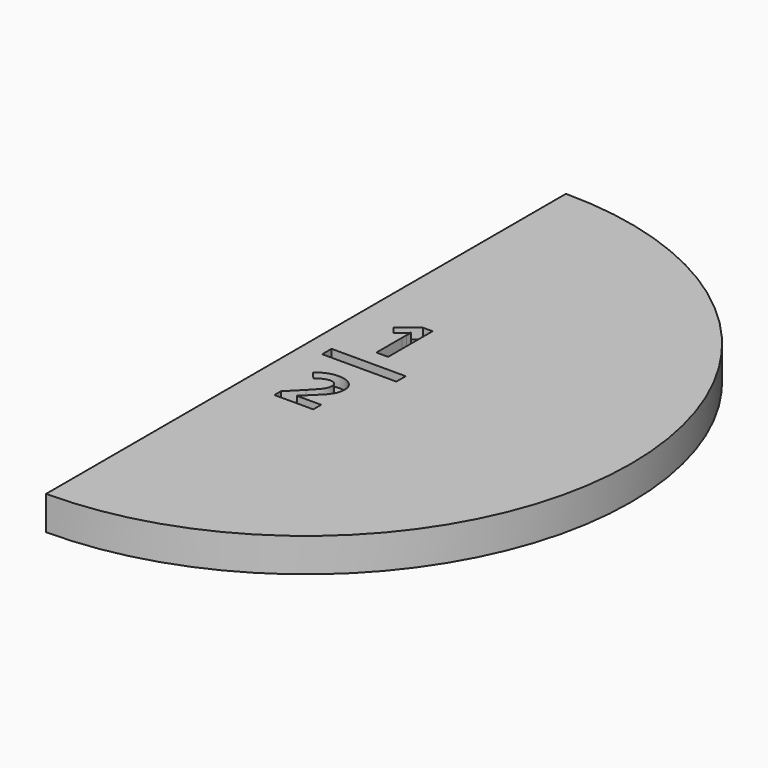
from build123d import *

# Parameters (mm, degrees)
F1_DEPTH      = 6.5
F2_R          = 12.5
F6_DEPTH      = 5
F3_R          = 12.5
F7_DEPTH      = 5
F4_R          = 12.5
F8_DEPTH      = 5
F5_R          = 12.5
F9_DEPTH      = 5
F10_W         = 14.2726595514
F10_H         = 2.253577346
F11_DEPTH     = 2
F15_TEXT_SIZE = 14.9677896982
F16_DEPTH     = 2


# Not quite as in the source:
# - Text() gives the source's letters only with a copy of the font that has no kerning and outlines rounded to 1/6400 em; it was checked with that copy


with BuildPart() as f1:
    # F0 (on Top) → F1 (new body)
    with BuildSketch(Plane.XY):
        with BuildLine():
            Line((0, 62.5), (0, -62.5))
            ThreePointArc((0, -62.5), (62.5, 0), (0, 62.5))
        make_face()
    extrude(amount=F1_DEPTH)

    # F2 (on face) → F6 (cut)
    with BuildSketch(Plane.XY.offset(6.5)):
        with Locations((17.2774232924, 41.4407812059)):
            Circle(F2_R)
    extrude(amount=-F6_DEPTH, mode=Mode.SUBTRACT)

    # F3 (on face) → F7 (cut)
    with BuildSketch(Plane.XY.offset(6.5)):
        with Locations((39.0620082617, 17.6530200988)):
            Circle(F3_R)
    extrude(amount=-F7_DEPTH, mode=Mode.SUBTRACT)

    # F4 (on face) → F8 (cut)
    with BuildSketch(Plane.XY.offset(6.5)):
        with Locations((41.0651862621, -17.6530200988)):
            Circle(F4_R)
    extrude(amount=-F8_DEPTH, mode=Mode.SUBTRACT)

    # F5 (on face) → F9 (cut)
    with BuildSketch(Plane.XY.offset(6.5)):
        with Locations((19.0302077681, -40.9399829805)):
            Circle(F5_R)
    extrude(amount=-F9_DEPTH, mode=Mode.SUBTRACT)

    # F10 (on face) → F11 (cut)
    with BuildSketch(Plane.XY):
        with Locations((11.1426881049, 0)):
            Rectangle(F10_W, F10_H)
    extrude(amount=F11_DEPTH, mode=Mode.SUBTRACT)


with BuildPart() as f13_1:
    # F13: instance of F1
    add(f1.part.mirror(Plane.XY))

    # F15 (on face) → F16 (cut)
    with BuildSketch(Plane.XY):
        with Locations((6.1007449403, 4.3819556013)):
            Text('1', F15_TEXT_SIZE, font='Open Sans', font_style=FontStyle.BOLD, text_align=(TextAlign.LEFT, TextAlign.BOTTOM))
        with Locations((6.1007449403, -15.9742383883)):
            Text('2', F15_TEXT_SIZE, font='Open Sans', font_style=FontStyle.BOLD, text_align=(TextAlign.LEFT, TextAlign.BOTTOM))
    extrude(amount=-F16_DEPTH, mode=Mode.SUBTRACT)


solid = f13_1.part
